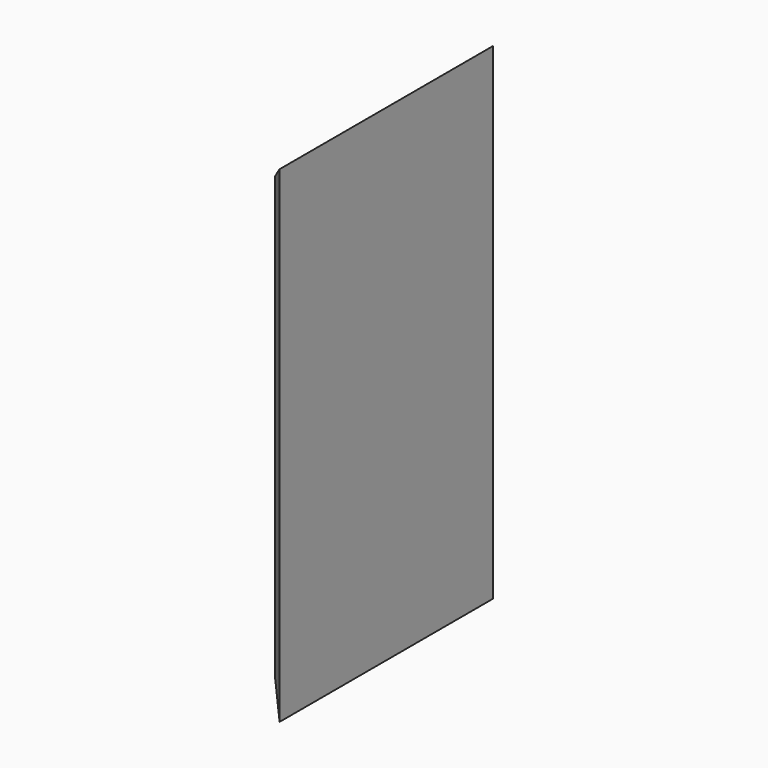
from build123d import *

# Parameters (mm, degrees)
F0_W     = 263
F0_H     = 480
F1_DEPTH = 22
F2_SIZE  = 21.99999


# Not quite as in the source:
# - a fillet or chamfer is up to 0.001 mm smaller than in the source, because OpenCascade refuses the exact size


with BuildPart() as f1:
    # F0 (on Right) → F1 (new body)
    with BuildSketch(Plane.YZ):
        Rectangle(F0_W, F0_H)
    extrude(amount=F1_DEPTH)

    # F2 (size 22 in the source; OpenCascade refuses exactly that, so slightly less here)
    f2_edges = [f1.edges().sort_by_distance(p)[0] for p in [
        (0, 131.5, 0),
        (0, 0, 240),
        (0, -131.5, 0),
        (0, 0, -240),
    ]]
    chamfer(f2_edges, length=F2_SIZE)


solid = f1.part
